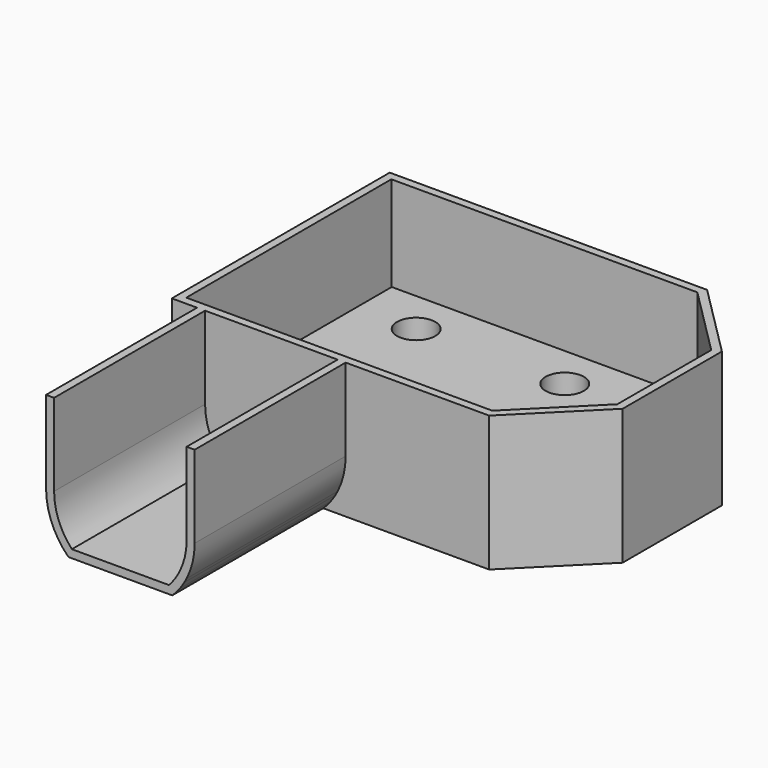
from build123d import *

# Parameters (mm, degrees)
F0_W     = 75.5
F0_H     = 62.83
F0_R     = 4.7625
F1_DEPTH = 10.5
F2_W     = 76.2071067812
F2_H     = 63.83
F3_DEPTH = 2
F4_DEPTH = 33.75
F9_DEPTH = 47


# Not quite as in the source:
# - a feature of the source that left no trace in its solid (it failed there, or was rolled back) is left out


with BuildPart() as f1:
    # F0 (on Top) → F1 (new body)
    with BuildSketch(Plane.XY):
        with Locations((-37.75, 31.415)):
            Rectangle(F0_W, F0_H)
        with Locations((-60.75, 10.83)):
            Circle(F0_R, mode=Mode.SUBTRACT)
        with Locations((-23.75, 10.83)):
            Circle(F0_R, mode=Mode.SUBTRACT)
        with Locations((-60.75, 52)):
            Circle(F0_R, mode=Mode.SUBTRACT)
        with Locations((-23.75, 52)):
            Circle(F0_R, mode=Mode.SUBTRACT)
        Polygon((0, 62.83), (0, 0), (17, 17), (17, 45.83), align=None)
    extrude(amount=F1_DEPTH)


with BuildPart() as f3:
    # F2 (on Top) → F3 (new body)
    with BuildSketch(Plane.XY):
        Polygon((1.0355339059, 0.3284271247), (0.2071067812, -0.5), (-76, -0.5), (-76, 63.33), (0.2071067812, 63.33), (1.0355339059, 62.5015728753), (1.0355339059, 65.33), (-78, 65.33), (-78, -2.5), (1.0355339059, -2.5), align=None)
        Polygon((17.5, 16.7928932188), (1.0355339059, 0.3284271247), (1.0355339059, -2.5), (19.5, 15.9644660941), (19.5, 46.8655339059), (1.0355339059, 65.33), (1.0355339059, 62.5015728753), (17.5, 46.0371067812), align=None)
        Polygon((1.0355339059, 62.5015728753), (1.0355339059, 0.3284271247), (17.5, 16.7928932188), (17.5, 46.0371067812), align=None)
        with Locations((-37.8964466094, 31.415)):
            Rectangle(F2_W, F2_H)
        Polygon((0.2071067812, 63.33), (0.2071067812, -0.5), (1.0355339059, 0.3284271247), (1.0355339059, 62.5015728753), align=None)
    extrude(amount=F3_DEPTH)

    # F2 (on Top) → F4 (join)
    with BuildSketch(Plane.XY):
        Polygon((1.0355339059, 0.3284271247), (0.2071067812, -0.5), (-76, -0.5), (-76, 63.33), (0.2071067812, 63.33), (1.0355339059, 62.5015728753), (1.0355339059, 65.33), (-78, 65.33), (-78, -2.5), (1.0355339059, -2.5), align=None)
        Polygon((17.5, 16.7928932188), (1.0355339059, 0.3284271247), (1.0355339059, -2.5), (19.5, 15.9644660941), (19.5, 46.8655339059), (1.0355339059, 65.33), (1.0355339059, 62.5015728753), (17.5, 46.0371067812), align=None)
    extrude(amount=F4_DEPTH)

    # F5: union 

    # F6 (on face) → F9 (join)
    with BuildSketch(Plane.XZ.offset(2.5)):
        with BuildLine():
            Line((-34.7144660941, 25.5687510354), (-34.7144660941, 28.1393741738))
            ThreePointArc((-34.7144660941, 28.1393741738), (-35.7447365731, 27.3232988085), (-36.7144660941, 26.4361342702))
            Line((-36.7144660941, 26.4361342702), (-36.7144660941, 23.4451856875))
            ThreePointArc((-36.7144660941, 23.4451856875), (-35.761487475, 24.5512536772), (-34.7144660941, 25.5687510354))
        make_face()
        with BuildLine():
            ThreePointArc((-36.7144660941, 26.4361342702), (-35.7447365731, 27.3232988085), (-34.7144660941, 28.1393741738))
            Line((-34.7144660941, 28.1393741738), (-34.7144660941, 33.75))
            Line((-34.7144660941, 33.75), (-36.7144660941, 33.75))
            Line((-36.7144660941, 33.75), (-36.7144660941, 26.4361342702))
        make_face()
        with BuildLine():
            Line((-34.7144660941, 13.2386868315), (-34.7144660941, 25.5687510354))
            ThreePointArc((-34.7144660941, 25.5687510354), (-35.761487475, 24.5512536772), (-36.7144660941, 23.4451856875))
            Line((-36.7144660941, 23.4451856875), (-36.7144660941, 21.6052870969))
            ThreePointArc((-36.7144660941, 21.6052870969), (-35.2214118786, 17.5398494651), (-34.7144660941, 13.2386868315))
        make_face()
        with BuildLine():
            ThreePointArc((-36.7144660941, 4.8720865662), (-35.2214118786, 8.937524198), (-34.7144660941, 13.2386868315))
            Line((-34.7144660941, 13.2386868315), (-36.7144660941, 13.2386868315))
            Line((-36.7144660941, 13.2386868315), (-36.7144660941, 4.8720865662))
        make_face()
        with BuildLine():
            Line((-36.7144660941, 13.2386868315), (-34.7144660941, 13.2386868315))
            ThreePointArc((-34.7144660941, 13.2386868315), (-35.2214118786, 17.5398494651), (-36.7144660941, 21.6052870969))
            Line((-36.7144660941, 21.6052870969), (-36.7144660941, 13.2386868315))
        make_face()
        with BuildLine():
            Line((-36.7144660941, 4.8720865662), (-36.7144660941, 13.2386868315))
            ThreePointArc((-36.7144660941, 13.2386868315), (-37.1624904325, 9.4197763374), (-38.482233047, 5.8082555219))
            ThreePointArc((-38.482233047, 5.8082555219), (-37.9233701313, 4.7908717814), (-37.2943615313, 3.8152972763))
            ThreePointArc((-37.2943615313, 3.8152972763), (-36.9958041312, 4.3389675026), (-36.7144660941, 4.8720865662))
        make_face()
        with BuildLine():
            ThreePointArc((-37.2943615313, 3.8152972763), (-37.9233701313, 4.7908717814), (-38.482233047, 5.8082555219))
            ThreePointArc((-38.482233047, 5.8082555219), (-39.0410959628, 4.7908717814), (-39.6701045628, 3.8152972763))
            ThreePointArc((-39.6701045628, 3.8152972763), (-39.1015956593, 2.9149999555), (-38.482233047, 2.0489008887))
            ThreePointArc((-38.482233047, 2.0489008887), (-37.8628704348, 2.9149999555), (-37.2943615313, 3.8152972763))
        make_face()
        with BuildLine():
            ThreePointArc((-40.25, 0.0412393929), (-39.3297816541, 1.0130769081), (-38.482233047, 2.0489008887))
            ThreePointArc((-38.482233047, 2.0489008887), (-39.1015956593, 2.9149999555), (-39.6701045628, 3.8152972763))
            ThreePointArc((-39.6701045628, 3.8152972763), (-39.9542699959, 3.4194608214), (-40.25, 3.0321879756))
            Line((-40.25, 3.0321879756), (-40.25, 0.0412393929))
        make_face()
        with BuildLine():
            ThreePointArc((-40.2921144901, 0), (-40.2710408208, 0.0206029237), (-40.25, 0.0412393929))
            Line((-40.25, 0.0412393929), (-40.25, 3.0321879756))
            ThreePointArc((-40.25, 3.0321879756), (-40.6812814796, 2.5069915592), (-41.1338237973, 2))
            ThreePointArc((-41.1338237973, 2), (-41.6789976888, 1.4411036608), (-42.25, 0.9086226277))
            Line((-42.25, 0.9086226277), (-42.25, 0))
            Line((-42.25, 0), (-40.2921144901, 0))
        make_face()
        with BuildLine():
            Line((-41.1338237973, 2), (-42.25, 2))
            Line((-42.25, 2), (-42.25, 0.9086226277))
            ThreePointArc((-42.25, 0.9086226277), (-41.6789976888, 1.4411036608), (-41.1338237973, 2))
        make_face()
        with BuildLine():
            Line((-42.25, 0.9086226277), (-42.25, 2))
            Line((-42.25, 2), (-65.2951083908, 2))
            ThreePointArc((-65.2951083908, 2), (-64.2243980751, 0.9492036132), (-63.0626725793, 0))
            Line((-63.0626725793, 0), (-60.75, 0))
            Line((-60.75, 0), (-43.3662596088, 0))
            ThreePointArc((-43.3662596088, 0), (-42.7982175494, 0.4421339263), (-42.25, 0.9086226277))
        make_face()
        with BuildLine():
            Line((-71.7144660941, 13.2386868315), (-69.7144660941, 13.2386868315))
            Line((-69.7144660941, 13.2386868544), (-69.7144660941, 21.6052870969))
            ThreePointArc((-69.7144660941, 21.6052870969), (-71.2075203095, 17.5398494651), (-71.7144660941, 13.2386868315))
        make_face()
        with BuildLine():
            ThreePointArc((-65.2951083908, 2), (-68.5699308893, 7.2004999412), (-69.7144660941, 13.2386868544))
            Line((-69.7144660941, 13.2386868544), (-69.7144660941, 4.8720865662))
            ThreePointArc((-69.7144660941, 4.8720865662), (-68.1259717308, 2.2889379921), (-66.136817698, 0))
            Line((-66.136817698, 0), (-63.0626725793, 0))
            ThreePointArc((-63.0626725793, 0), (-64.2243980751, 0.9492036132), (-65.2951083908, 2))
        make_face()
        with BuildLine():
            Line((-69.7144660941, 4.8720865662), (-69.7144660941, 13.2386868544))
            Line((-69.7144660941, 13.2386868315), (-71.7144660941, 13.2386868315))
            ThreePointArc((-71.7144660941, 13.2386868315), (-71.2075203095, 8.937524198), (-69.7144660941, 4.8720865662))
        make_face()
        with BuildLine():
            ThreePointArc((-71.7144660941, 13.2386868315), (-71.2075203095, 17.5398494651), (-69.7144660941, 21.6052870969))
            Line((-69.7144660941, 21.6052870969), (-69.7144660941, 33.75))
            Line((-69.7144660941, 33.75), (-71.7144660941, 33.75))
            Line((-71.7144660941, 33.75), (-71.7144660941, 13.2386868315))
        make_face()
        with BuildLine():
            Line((-43.3662596088, 0), (-42.25, 0))
            Line((-42.25, 0), (-42.25, 0.9086226277))
            ThreePointArc((-42.25, 0.9086226277), (-42.7982175494, 0.4421339263), (-43.3662596088, 0))
        make_face()
    extrude(amount=F9_DEPTH)


solid = Compound([f1.part, f3.part])
